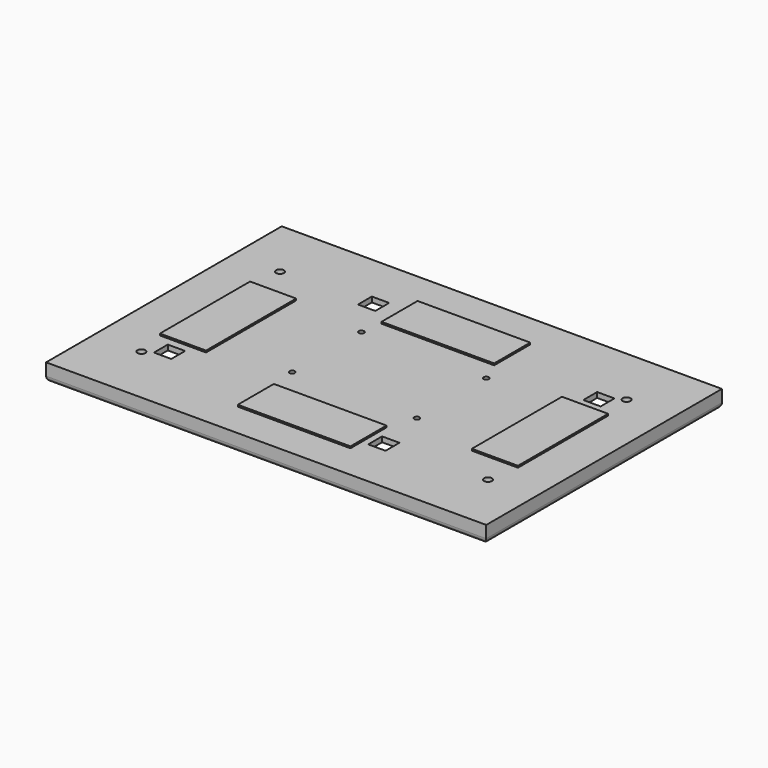
from build123d import *

# Parameters (mm, degrees)
F0_W      = 254
F0_H      = 170
F0_R      = 2.2742272187
F1_DEPTH  = 3
F2_W      = 254
F2_H      = 170
F2_W_2    = 238
F2_H_2    = 150
F3_DEPTH  = 10
F4_R      = 3
F5_R      = 1.5
F6_DEPTH  = 25
F7_W      = 26.6
F7_H      = 65
F7_W_2    = 65
F7_H_2    = 26
F8_DEPTH  = 1
F9_W      = 10
F9_H      = 10
F10_DEPTH = 25


# Not quite as in the source:
# - a feature names something its author has since deleted; it is built from what else it names


with BuildPart() as f1:
    # F0 (on Top) → F1 (new body)
    with BuildSketch(Plane.XY):
        Rectangle(F0_W, F0_H)
        with Locations((-100, -50)):
            Circle(F0_R, mode=Mode.SUBTRACT)
        with Locations((100, -50)):
            Circle(F0_R, mode=Mode.SUBTRACT)
        with Locations((-100, 50)):
            Circle(F0_R, mode=Mode.SUBTRACT)
        with Locations((100, 50)):
            Circle(F0_R, mode=Mode.SUBTRACT)
    extrude(amount=F1_DEPTH)

    # F2 (on face) → F3 (join)
    with BuildSketch(Plane.XY.offset(3)):
        Rectangle(F2_W, F2_H)
        Rectangle(F2_W_2, F2_H_2, mode=Mode.SUBTRACT)
    extrude(amount=-F3_DEPTH)

    # F4
    f4_edges = [f1.edges().sort_by_distance(p)[0] for p in [
        (-127, 0, -7),
        (-119, 0, -7),
        (0, 75, -7),
        (0, 85, -7),
        (119, 0, -7),
        (127, 0, -7),
        (0, -75, -7),
        (0, -85, -7),
    ]]
    fillet(f4_edges, radius=F4_R)

    # F5 (on face) → F6 (cut)
    with BuildSketch(Plane.XY.offset(3)):
        with Locations((-34.4810113311, -23.1507848948)):
            Circle(F5_R)
        with Locations((-34.4810113311, 26.8492151052)):
            Circle(F5_R)
        with Locations((37.5189886689, -23.1507848948)):
            Circle(F5_R)
        with Locations((37.5189886689, 26.8492151052)):
            Circle(F5_R)
    extrude(amount=-F6_DEPTH, mode=Mode.SUBTRACT)

    # F7 (on face) → F8 (join)
    with BuildSketch(Plane.XY.offset(3)):
        with Locations((-90, 0)):
            Rectangle(F7_W, F7_H)
        with Locations((0, 51.8365384532)):
            Rectangle(F7_W_2, F7_H_2)
        with Locations((0, -51.8365384532)):
            Rectangle(F7_W_2, F7_H_2)
        with Locations((90, 0)):
            Rectangle(F7_W, F7_H)
    extrude(amount=F8_DEPTH)

    # F9 (on face) → F10 (cut)
    with BuildSketch(Plane.XY.offset(3)):
        with Locations((-47.5, 51.8365384532)):
            Rectangle(F9_W, F9_H)
        with Locations((90, 42.4970947206)):
            Rectangle(F9_W, F9_H)
        with Locations((41.3667224348, -51.8365384532)):
            Rectangle(F9_W, F9_H)
        with Locations((-90, -42.1905592084)):
            Rectangle(F9_W, F9_H)
    extrude(amount=-F10_DEPTH, mode=Mode.SUBTRACT)


solid = f1.part
